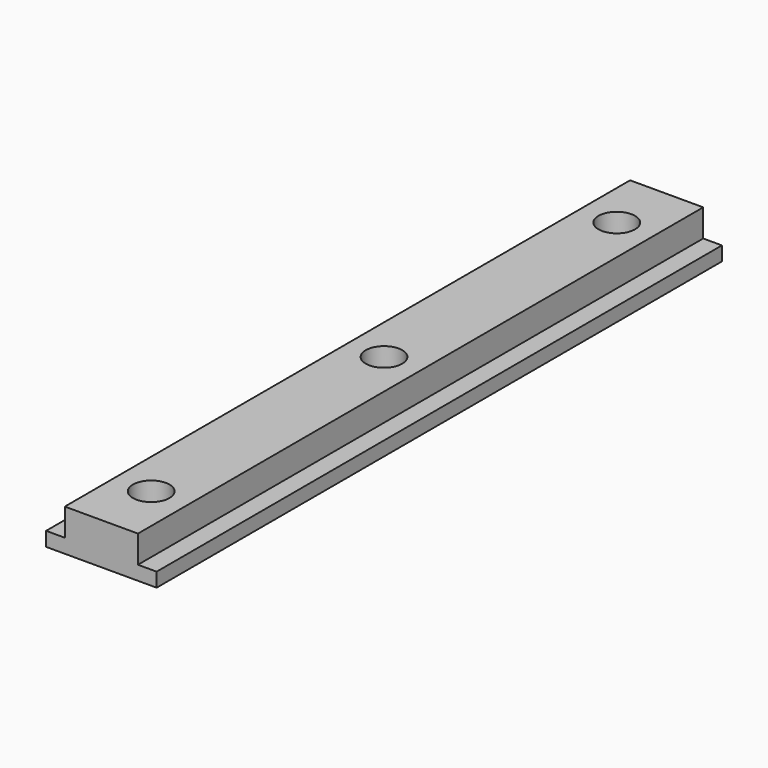
from build123d import *

# Parameters (mm, degrees)
F0_W           = 8.8
F0_H           = 3.3
F1_DEPTH       = 42.5
F3_D           = 4.4
F3_CSINK_D     = 8.96
F3_CSINK_ANGLE = 90


with BuildPart() as f1:
    # F0 (on Front) → F1 (new body, symmetric)
    with BuildSketch(Plane.XZ):
        Polygon((6.65, -0.85), (6.65, 0.85), (4.4, 0.85), (-4.4, 0.85), (-6.65, 0.85), (-6.65, -0.85), align=None)
        with Locations((0, 2.5)):
            Rectangle(F0_W, F0_H)
    extrude(amount=F1_DEPTH, both=True)

    # F3 (through all)
    with Locations(Plane(origin=(0, 0, -0.85), x_dir=(1, 0, 0), z_dir=(0, 0, -1))):
        with Locations((0, -35), (0, 0), (0, 35)):
            CounterSinkHole(F3_D / 2, F3_CSINK_D / 2, counter_sink_angle=F3_CSINK_ANGLE)


solid = f1.part
